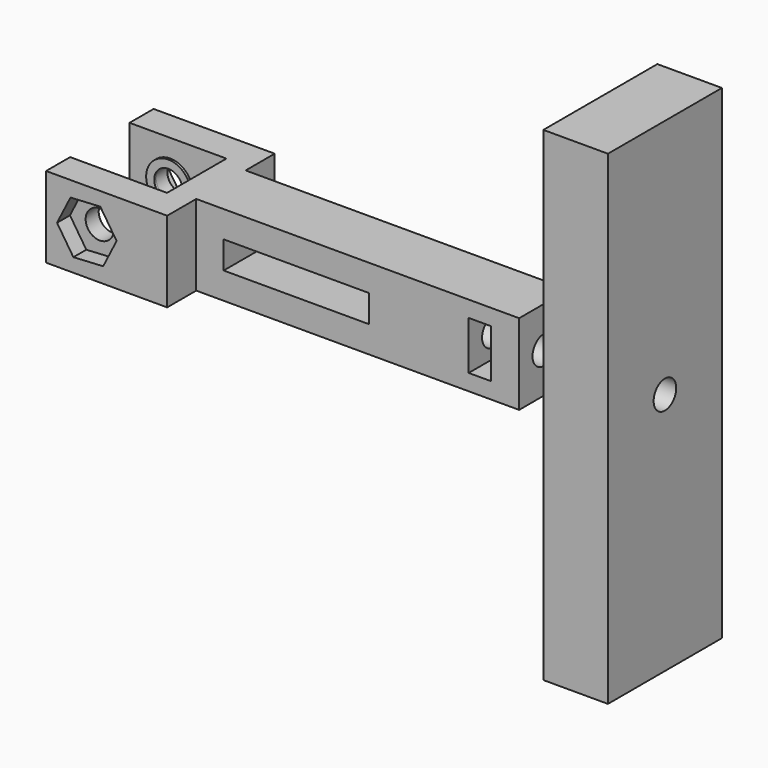
from build123d import *

# Parameters (mm, degrees)
F0_W      = 40
F0_H      = 3.825
F1_DEPTH  = 10
F2_R      = 1.75
F3_DEPTH  = 16.651
F4_W      = 18
F4_H      = 3.4
F4_W_2    = 2.75
F4_H_2    = 6
F5_DEPTH  = 12.151
F6_R      = 1.75
F7_DEPTH  = 15
F10_DEPTH = 2
F11_W     = 17.65
F11_H     = 60
F12_DEPTH = 8
F13_R     = 1.75
F14_DEPTH = 70.001
F15_R     = 2.75
F15_R_2   = 1.75
F16_DEPTH = 0.3
F17_R     = 1.75
F18_DEPTH = 2
F19_R     = 3.75
F20_DEPTH = 1


# Not quite as in the source:
# - a pattern or mirror of a feature is missing from the dataset's text; its kind, count and spacing are read off the source's solid


with BuildPart() as f1:
    # F0 (on Top) → F1 (new body)
    with BuildSketch(Plane.XY):
        Polygon((0, -3.825), (0, 0), (-3, 0), (-3, -4.6), (-15, -4.6), (-15, -8.325), (0, -8.325), align=None)
        Polygon((-3, 0), (0, 0), (0, 3.825), (0, 8.325), (-15, 8.325), (-15, 4.6), (-3, 4.6), align=None)
        with Locations((20, 1.9125)):
            Rectangle(F0_W, F0_H)
        with Locations((20, -1.9125)):
            Rectangle(F0_W, F0_H)
    extrude(amount=F1_DEPTH)

    # F2 (on face) → F3 (cut, through all)
    with BuildSketch(Plane.XZ.offset(8.325)):
        with Locations((-9.9527407438, 5)):
            Circle(F2_R)
    extrude(amount=-F3_DEPTH, mode=Mode.SUBTRACT)

    # F4 (on face) → F5 (cut, through all)
    with BuildSketch(Plane.XZ.offset(3.825)):
        with Locations((12.4002694301, 5)):
            Rectangle(F4_W, F4_H)
        with Locations((35.125, 5)):
            Rectangle(F4_W_2, F4_H_2)
    extrude(amount=-F5_DEPTH, mode=Mode.SUBTRACT)

    # F6 (on face) → F7 (cut)
    with BuildSketch(Plane.YZ.offset(40)):
        with Locations((0, 5)):
            Circle(F6_R)
    extrude(amount=-F7_DEPTH, mode=Mode.SUBTRACT)

    # F15 (on face) → F16 (join)
    with BuildSketch(Plane.XZ.offset(-4.6)):
        with Locations((-9.9527407438, 5)):
            Circle(F15_R)
        with Locations((-9.9527407438, 5)):
            Circle(F15_R_2, mode=Mode.SUBTRACT)
    f16 = extrude(amount=F16_DEPTH)

    # F16_copies: F16 across plane
    add(f16.mirror(Plane(origin=(0, 0, 0), x_dir=(0, 0, -1), z_dir=(0, -1, 0))))

    # F17 (on face) → F18 (cut)
    with BuildSketch(Plane.XZ.offset(8.325)):
        Polygon((-7.9284293953, 1.9088033227), (-6.2635302189, 5.2075067143), (-8.2878415673, 8.2987033916), (-11.9770520922, 8.0911966773), (-13.6419512686, 4.7924932857), (-11.6176399202, 1.7012966084), align=None)
        with Locations((-9.9527407438, 5)):
            Circle(F17_R, mode=Mode.SUBTRACT)
    f18 = extrude(amount=-F18_DEPTH, mode=Mode.SUBTRACT)

    # F18_copies: F18 across plane
    add(f18.mirror(Plane.ZX), mode=Mode.SUBTRACT)


with BuildPart() as f10:
    # F9 (on offset) → F10 (new body)
    with BuildSketch(Plane.YZ.offset(45)):
        Polygon((3.825, 0), (3.825, 10), (3.825, 19.8484882712), (-3.825, 19.8484882712), (-3.825, 10), (-3.825, 0), (-3.825, -10.1515117288), (3.825, -10.1515117288), align=None)
    extrude(amount=F10_DEPTH)

    # F11 (on face) → F12 (join)
    with BuildSketch(Plane.YZ.offset(47)):
        with Locations((0, 4.8484882712)):
            Rectangle(F11_W, F11_H)
    extrude(amount=F12_DEPTH)

    # F13 (on face) → F14 (cut, through all)
    with BuildSketch(Plane.YZ.offset(55)):
        with Locations((0, 5)):
            Circle(F13_R)
    extrude(amount=-F14_DEPTH, mode=Mode.SUBTRACT)

    # F19 (on face) → F20 (join)
    with BuildSketch(Plane(origin=(47, 0, 0), x_dir=(0, -1, 0), z_dir=(-1, 0, 0))):
        with Locations((0, 28)):
            Circle(F19_R)
        with Locations((0, -18)):
            Circle(F19_R)
    extrude(amount=F20_DEPTH)


solid = Compound([f1.part, f10.part])
